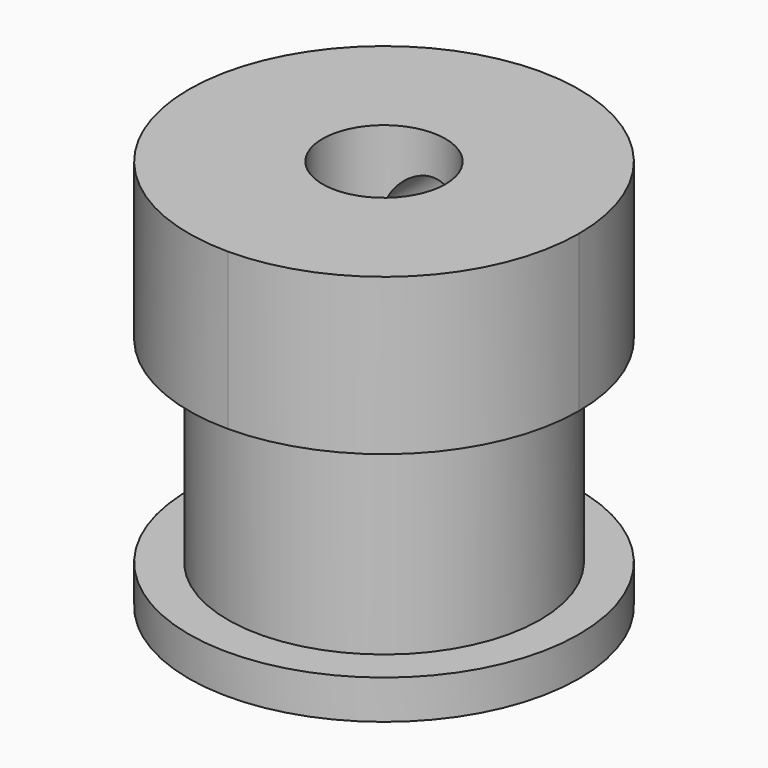
from build123d import *

# Parameters (mm, degrees)
F0_R         = 7.9375
F1_DEPTH     = 1.5875
F2_R         = 6.35
F3_DEPTH     = 8
F4_W         = 15.875
F4_H         = 15.875
F5_DEPTH     = 6.35
F6_R         = 2.5
F7_DEPTH     = 15.9375
F8_R         = 1.5875
F9_REACH     = 20.3661280605
F10_T1_DEPTH = 46.0375
F11_R        = 4.0875
F11_R_2      = 2.5
F12_DEPTH    = 1.5875


# Not quite as in the source:
# - a fillet or chamfer that OpenCascade refuses, or shapes differently, is made with other operations: its cross-section is extruded or revolved along the edge and cut away or added


with BuildPart() as f1:
    # F0 (on Top) → F1 (new body)
    with BuildSketch(Plane.XY):
        Circle(F0_R)
    extrude(amount=F1_DEPTH)

    # F2 (on face) → F3 (join)
    with BuildSketch(Plane.XY.offset(1.5875)):
        Circle(F2_R)
    extrude(amount=F3_DEPTH)

    # F4 (on face) → F5 (join)
    with BuildSketch(Plane.XY.offset(9.5875)):
        Rectangle(F4_W, F4_H)
    extrude(amount=F5_DEPTH)

    # F6 (on face) → F7 (cut, through all)
    with BuildSketch(Plane.XY.offset(15.9375)):
        Circle(F6_R)
    extrude(amount=-F7_DEPTH, mode=Mode.SUBTRACT)

    f9_end = f1.faces().sort_by_distance((-2.5, 0, 7.96875))[0]
    # F8 (on face) → F9 (cut, up to a face of the model that its end follows)
    with BuildSketch(Plane(origin=(0, 7.9375, 0), x_dir=(-1, 0, 0), z_dir=(0, 1, 0))):
        with Locations((0, 12.7625)):
            Circle(F8_R)
    f9_long = extrude(amount=-F9_REACH, mode=Mode.PRIVATE)
    add(split(f9_long, bisect_by=f9_end, keep=Keep.ALL, mode=Mode.PRIVATE).solids().sort_by_distance((0, 7.9375, 12.7625))[0], mode=Mode.SUBTRACT)

    # F10: fillet of radius 7.9375 on 4 edges, made by hand

    # F10_s2 → F10_t1 (cut)
    with BuildSketch(Plane.XY.offset(-10.25625)):
        with BuildLine():
            ThreePointArc((-7.9375, 0), (-5.6126600757, 5.6126600757), (0, 7.9375))
            Line((0, 7.9375), (-7.9375, 7.9375))
            Line((-7.9375, 7.9375), (-7.9375, 0))
        make_face()
        with BuildLine():
            ThreePointArc((0, -7.9375), (-5.6126600757, -5.6126600757), (-7.9375, 0))
            Line((-7.9375, 0), (-7.9375, -7.9375))
            Line((-7.9375, -7.9375), (0, -7.9375))
        make_face()
        with BuildLine():
            ThreePointArc((7.9375, 0), (5.6126600757, 5.6126600757), (0, 7.9375))
            Line((0, 7.9375), (7.9375, 7.9375))
            Line((7.9375, 7.9375), (7.9375, 0))
        make_face()
        with BuildLine():
            ThreePointArc((0, -7.9375), (5.6126600757, -5.6126600757), (7.9375, 0))
            Line((7.9375, 0), (7.9375, -7.9375))
            Line((7.9375, -7.9375), (0, -7.9375))
        make_face()
    extrude(amount=F10_T1_DEPTH, mode=Mode.SUBTRACT)

    # F11 (on face) → F12 (join)
    with BuildSketch(Plane(origin=(0, 0, 0), x_dir=(1, 0, 0), z_dir=(0, 0, -1))):
        Circle(F11_R)
        Circle(F11_R_2, mode=Mode.SUBTRACT)
    extrude(amount=F12_DEPTH)


solid = f1.part
